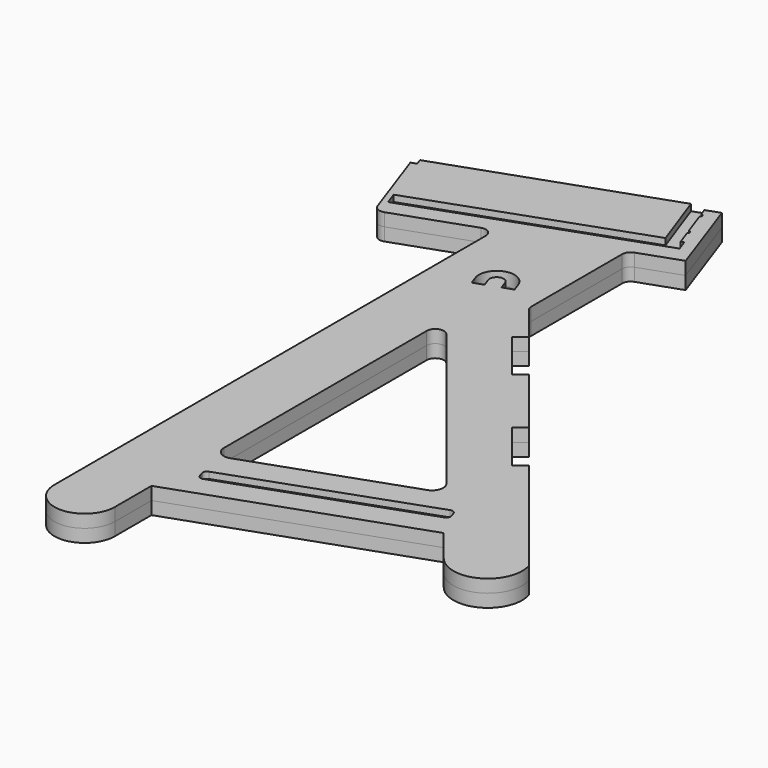
from build123d import *

# Parameters (mm, degrees)
F1_DEPTH = 19.05
F3_DEPTH = 9.525
F5_DEPTH = 9.525
F6_W     = 94.742
F6_H     = 19.05
F6_H_2   = 22.0252738774
F7_DEPTH = 19.558
F8_R     = 3.302
F9_DEPTH = 19.051


# Not quite as in the source:
# - ends of sketch curves that miss each other by under 0.0002 mm in the source are joined
# - a feature names something its author has since deleted; it is built from what else it names
# - the program builds the solid bodies; features that only make, move or delete a surface that nothing else refers to are left out


with BuildPart() as f1:
    # F0 (on Top) → F1 (new body)
    with BuildSketch(Plane.XY):
        with BuildLine():
            Line((727.2677384075, 507.6293858847), (727.2677384075, -289.3185215378))
            ThreePointArc((727.2677384075, -289.3185215378), (771.8616098047, -333.912392935), (816.4554812019, -289.3185215378))
            Line((816.4554812019, -289.3185215378), (816.4554812019, -221.6290421598))
            Line((816.4554812019, -221.6290421598), (1153.5588304871, -102.9697649078))
            Line((1153.5588304871, -102.9697649078), (1192.9737952894, -152.2336658633))
            ThreePointArc((1192.9737952894, -152.2336658633), (1256.5580507142, -165.3785793409), (1281.2649482254, -105.3342998163))
            Line((1281.2649482254, -105.3342998163), (881.6774022659, 394.10141923))
            ThreePointArc((881.6774022659, 394.10141923), (879.6100790274, 397.83144491), (878.8940586752, 402.0355181492))
            Line((878.8940586752, 402.0355181492), (878.8940586752, 569.9420720746))
            ThreePointArc((878.8940586752, 569.9420720746), (881.2296299338, 577.2815963686), (887.3773054254, 581.9215959395))
            Line((887.3773054254, 581.9215959395), (946.5202680448, 602.7397254948))
            Line((946.5202680448, 602.7397254948), (904.3527355464, 722.5349641439))
            Line((904.3527355464, 722.5349641439), (884.020881133, 715.3782178375))
            Line((884.020881133, 715.3782178375), (880.8583161956, 724.3628607361))
            Line((880.8583161956, 724.3628607361), (549.7442765696, 607.8118009104))
            Line((549.7442765696, 607.8118009104), (552.906841507, 598.8271580117))
            Line((552.906841507, 598.8271580117), (544.9670195991, 596.0323666485))
            Line((544.9670195991, 596.0323666485), (582.9177988478, 488.2166518643))
            ThreePointArc((582.9177988478, 488.2166518643), (589.40821497, 480.9809077363), (599.1140759625, 480.4538812492))
            Line((599.1140759625, 480.4538812492), (710.3509851577, 519.6089097496))
            ThreePointArc((710.3509851577, 519.6089097497), (721.9072627016, 517.9938146262), (727.2677384075, 507.6293858847))
        make_face()
        with BuildLine():
            ThreePointArc((844.5095176323, -110.7755588107), (829.4863568252, -108.6759351502), (822.5177384075, -95.2021777863))
            Line((822.5177384075, -95.2021777863), (822.5177384075, 279.3762959499))
            ThreePointArc((822.5177384075, 279.3762959499), (831.0136651683, 291.3602755977), (845.1343948168, 287.3103948691))
            Line((845.1343948168, 287.3103948691), (1078.976974464, -4.9643221252))
            ThreePointArc((1078.976974464, -4.9643221252), (1081.9579117622, -19.8218837855), (1071.5671003568, -30.8520317446))
            Line((1071.5671003568, -30.8520317446), (844.5095176323, -110.7755588107))
        make_face(mode=Mode.SUBTRACT)
        with BuildLine():
            Line((822.1982316908, 418.0308171084), (817.981478441, 430.0103409733))
            ThreePointArc((817.981478441, 430.0103409733), (804.7653209472, 436.3447634256), (798.4309001253, 423.1286012999))
            Line((798.4309001253, 423.1286012999), (802.6476533752, 411.149077435))
            Line((802.6476533752, 411.149077435), (787.6732485441, 405.8781358727))
            Line((787.6732485441, 405.8781358727), (783.4564952942, 417.8576597376))
            ThreePointArc((783.4564952942, 417.8576597376), (799.4943781806, 451.3191657439), (832.9558841868, 435.2812828576))
            Line((832.9558841868, 435.2812828576), (837.1726374367, 423.3017589927))
            Line((837.1726374367, 423.3017589927), (822.1982316908, 418.0308171084))
        make_face(mode=Mode.SUBTRACT)
    extrude(amount=F1_DEPTH)

    # F2 (on face) → F3 (cut)
    with BuildSketch(Plane.XY):
        with BuildLine():
            ThreePointArc((844.1222933391, -166.9052020902), (847.3560158569, -170.6500208272), (852.2954479263, -170.9374917442))
            Line((852.2954479263, -170.9374917442), (1129.8610507564, -72.1108335167))
            ThreePointArc((1129.8610507564, -72.1108335167), (1133.425786756, -68.9382065458), (1133.77435322, -64.1788572139))
            Line((1133.77435322, -64.1788572139), (1131.667577719, -57.6492424267))
            ThreePointArc((1131.667577719, -57.6492424267), (1128.4338552012, -53.9044236898), (1123.4944231318, -53.6169527728))
            Line((1123.4944231318, -53.6169527728), (845.9288203018, -152.4436110002))
            ThreePointArc((845.9288203018, -152.4436110002), (842.3640843021, -155.6162379711), (842.0155178382, -160.3755873031))
            Line((842.0155178382, -160.3755873031), (844.1222933391, -166.9052020902))
        make_face()
    extrude(amount=F3_DEPTH, mode=Mode.SUBTRACT)

    # F4 (on face) → F5 (cut)
    with BuildSketch(Plane.XY):
        Polygon((579.9443241227, 521.366756094), (586.5044770697, 502.9417796404), (921.8787370542, 622.3506942479), (916.3315891482, 637.930524532), (912.1286802344, 636.4340924814), (884.020881133, 715.3782178375), (880.8583161956, 724.3628607361), (862.3802941818, 717.9536434315), (892.7236092325, 632.7308033777), align=None)
    extrude(amount=F5_DEPTH, mode=Mode.SUBTRACT)

    # F6 (on face) → F7 (cut)
    with BuildSketch(Plane(origin=(729.8159568657, 583.9097126711, 0), x_dir=(-0.6247321984, 0.7808390873, 0), z_dir=(0.7808390873, 0.6247321984, 0))):
        with Locations((-357.8801403508, 9.525)):
            Rectangle(F6_W, F6_H)
        with Locations((-584.9891603508, 10.3152221296)):
            Rectangle(F6_W, F6_H_2)
    extrude(amount=-F7_DEPTH, mode=Mode.SUBTRACT)

    # F8 (on face) → F9 (cut, through all)
    with BuildSketch(Plane.XY):
        with BuildLine():
            ThreePointArc((902.3498094673, 663.8992240234), (899.5515171423, 659.5044786379), (904.4975380125, 657.8670707805))
            Line((904.4975380125, 657.8670707805), (902.3498094673, 663.8992240234))
        make_face()
        with BuildLine():
            ThreePointArc((887.5764301968, 705.3920317976), (884.8076232072, 701.0002222812), (889.7289379426, 699.3464555963))
            Line((889.7289379426, 699.3464555963), (887.5764301968, 705.3920317976))
        make_face()
        with BuildLine():
            Line((887.5764301968, 705.3920317976), (889.7289379426, 699.3464555963))
            ThreePointArc((889.7289379426, 699.3464555963), (890.8236579238, 700.5386106968), (891.2203335175, 702.107780571))
            ThreePointArc((891.2203335175, 702.107780571), (890.1290165833, 704.5605513272), (887.5764301968, 705.3920317976))
        make_face()
        with BuildLine():
            Line((902.3498094673, 663.8992240234), (904.4975380125, 657.8670707805))
            ThreePointArc((904.4975380125, 657.8670707805), (905.5745632393, 659.0559185948), (905.9642274527, 660.6120369276))
            ThreePointArc((905.9642274527, 660.6120369276), (904.8838934731, 663.0548639976), (902.3498094673, 663.8992240234))
        make_face()
        with Locations((880.5389518172, 617.9122097817)):
            Circle(F8_R)
        with BuildLine():
            ThreePointArc((623.7483495144, 526.4827509324), (617.3838130375, 524.8132146381), (623.9396392041, 525.3751926427))
            ThreePointArc((623.9396392041, 525.3751926427), (623.8914653707, 525.9371706472), (623.7483495144, 526.4827509324))
        make_face()
        with BuildLine():
            ThreePointArc((756.0284718398, 572.4049919407), (752.1644938352, 575.6588181073), (749.6157615295, 571.2974336509))
            ThreePointArc((749.6157615295, 571.2974336509), (753.2884498444, 569.1511657741), (756.0284718398, 572.4049919407))
        make_face()
        with Locations((1055.4790926394, -88.2571151612)):
            Circle(F8_R)
        with Locations((913.5925848765, -138.7755124943)):
            Circle(F8_R)
    extrude(amount=F9_DEPTH, mode=Mode.SUBTRACT)


with BuildPart() as f12_1:
    # F12: instance of F1
    add(f1.part.mirror(Plane.XY.offset(19.05)))


solid = Compound([f1.part, f12_1.part])
